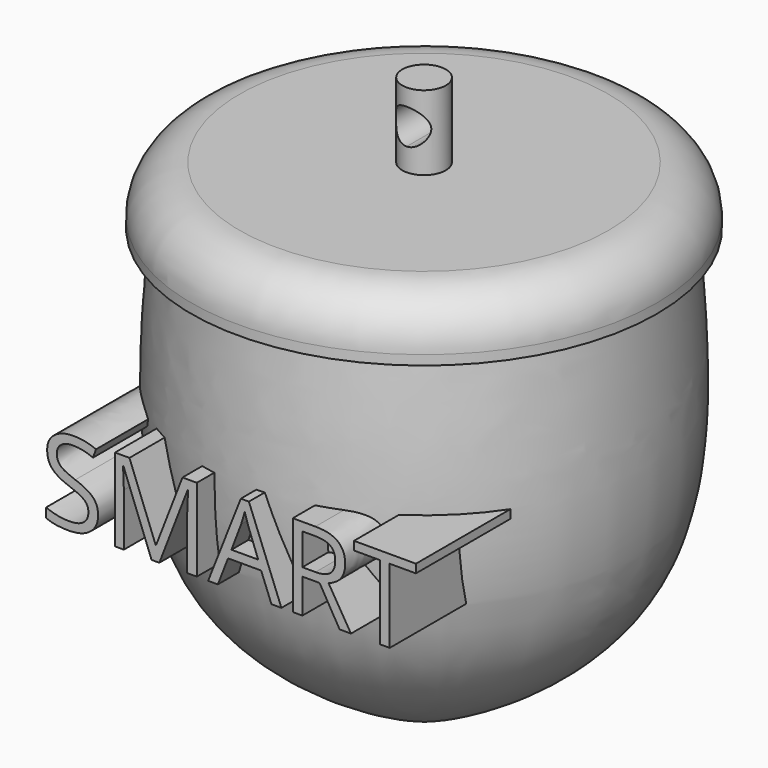
from build123d import *

# Parameters (mm, degrees)
F2_TEXT_SIZE   = 12.199881
F3_DEPTH       = 25.4
F4_R           = 24.528001
F5_DEPTH       = 6.096
F6_R           = 5.08
F7_R           = 2.29543
F8_DEPTH       = 7.874
F10_DEPTH      = 17.526
F10_DEPTH_BACK = 25.4


# Not quite as in the source:
# - Text() gives the source's letters only with a copy of the font that has no kerning and outlines rounded to 1/6400 em; it was checked with that copy


with BuildPart() as f1:
    # F0 (on Front) → F1 (revolve)
    with BuildSketch(Plane.XZ):
        with BuildLine():
            Line((0, -45.733642), (0, 0))
            add(Edge.make_bspline(
                [(0, 0), (-7.542709, 0), (-15.085418, 0), (-22.628127, 0)],
                knots=[0, 0, 0, 0, 22.628127, 22.628127, 22.628127, 22.628127], degree=3))
            add(Edge.make_bspline(
                [(-22.628127, 0), (-23.531902, -11.438826), (-25.253332, -33.226494), (-8.132269, -41.705995), (0, -45.733642)],
                knots=[0, 0, 0, 0, 0.525014, 1, 1, 1, 1], degree=3))
        make_face()
    revolve(axis=Axis((0, 0, -22.866821), (0, 0, -1)))

    # F2 (on Front) → F3 (join)
    with BuildSketch(Plane.XZ):
        with Locations((-20.145717, -23.200985)):
            Text('SMART', F2_TEXT_SIZE, font='Open Sans', text_align=(TextAlign.LEFT, TextAlign.BOTTOM))
    extrude(amount=F3_DEPTH)

    # F4 (on face) → F5 (join)
    with BuildSketch(Plane.XY):
        Circle(F4_R)
    extrude(amount=F5_DEPTH)

    # F6
    f6_edges = [f1.edges().sort_by_distance(p)[0] for p in [
        (-24.528001, 0, 6.096),
    ]]
    fillet(f6_edges, radius=F6_R)

    # F7 (on face) → F8 (join)
    with BuildSketch(Plane.XY.offset(6.096)):
        Circle(F7_R)
    extrude(amount=F8_DEPTH)

    # F9 (on Front) → F10 (cut, two sides)
    with BuildSketch(Plane.XZ) as f10_sk:
        with BuildLine():
            ThreePointArc((0, 12.194), (-1.850502, 10.343499), (0, 8.492997))
            Line((0, 8.492997), (0, 12.194))
        make_face()
        with BuildLine():
            Line((0, 12.194), (0, 8.492997))
            ThreePointArc((0, 8.492997), (1.308502, 9.034996), (1.850502, 10.343499))
            ThreePointArc((1.850502, 10.343499), (1.308502, 11.652001), (0, 12.194))
        make_face()
    extrude(amount=F10_DEPTH, mode=Mode.SUBTRACT)
    extrude(f10_sk.sketch, amount=-F10_DEPTH_BACK, mode=Mode.SUBTRACT)


solid = f1.part
